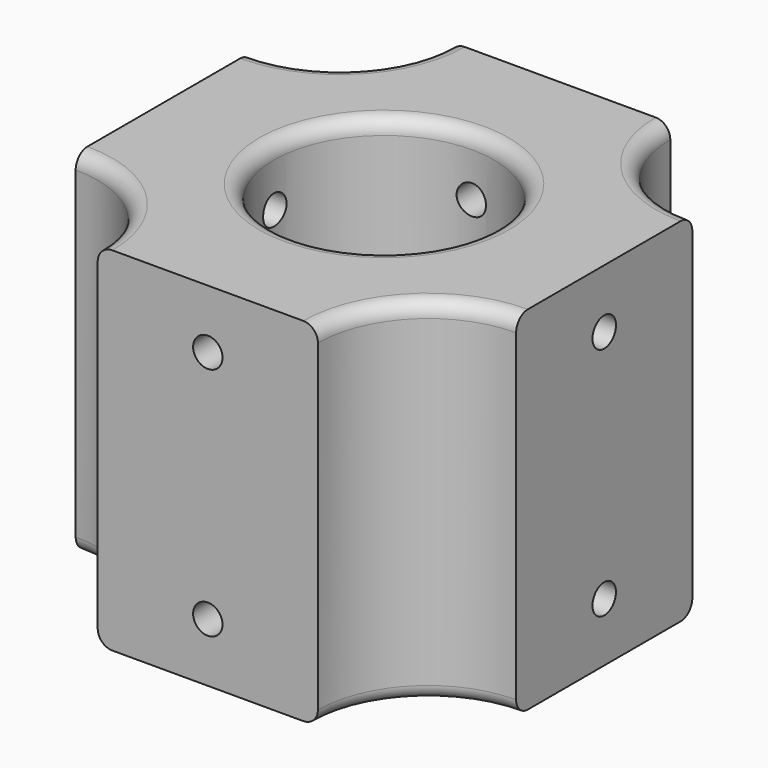
from build123d import *

# Parameters (mm, degrees)
F0_W     = 15
F0_H     = 7.5
F0_W_2   = 7.5
F0_H_2   = 15
F1_DEPTH = 12
F3_D     = 2
F5_D     = 15
F7_D     = 2
F8_R     = 1


with BuildPart() as f1:
    # F0 (on Top) → F1 (new body, symmetric)
    with BuildSketch(Plane.XY):
        with BuildLine():
            Line((-15, 7.5), (-7.5, 7.5))
            Line((-7.5, 7.5), (-7.5, 15))
            ThreePointArc((-7.5, 15), (-9.6966991411, 9.6966991411), (-15, 7.5))
        make_face()
        with Locations((0, 11.25)):
            Rectangle(F0_W, F0_H)
        with BuildLine():
            Line((7.5, 7.5), (15, 7.5))
            ThreePointArc((15, 7.5), (9.6966991411, 9.6966991411), (7.5, 15))
            Line((7.5, 15), (7.5, 7.5))
        make_face()
        with Locations((11.25, 0)):
            Rectangle(F0_W_2, F0_H_2)
        with Locations((0, -11.25)):
            Rectangle(F0_W, F0_H)
        with BuildLine():
            ThreePointArc((7.5, -15), (9.6966991411, -9.6966991411), (15, -7.5))
            Line((15, -7.5), (7.5, -7.5))
            Line((7.5, -7.5), (7.5, -15))
        make_face()
        with BuildLine():
            Line((-7.5, -15), (-7.5, -7.5))
            Line((-7.5, -7.5), (-15, -7.5))
            ThreePointArc((-15, -7.5), (-9.6966991411, -9.6966991411), (-7.5, -15))
        make_face()
        with Locations((-11.25, 0)):
            Rectangle(F0_W_2, F0_H_2)
        Rectangle(F0_W, F0_H_2)
    extrude(amount=F1_DEPTH, both=True)

    # F3 (through all)
    with Locations(Plane.XZ.offset(15)):
        with Locations((0, 8), (0, -8)):
            Hole(F3_D / 2)

    # F5 (through all)
    with Locations(Plane.XY.offset(12)):
        with Locations((0, 0)):
            Hole(F5_D / 2)

    # F7 (through all)
    with Locations(Plane(origin=(-15, 0, 0), x_dir=(0, -1, 0), z_dir=(-1, 0, 0))):
        with Locations((0, -8), (0, 8)):
            Hole(F7_D / 2)

    # F8
    f8_edges = [f1.edges().sort_by_distance(p)[0] for p in [
        (-9.696699, 9.696699, 12),
        (-9.696699, -9.696699, 12),
        (9.696699, -9.696699, 12),
        (9.696699, 9.696699, 12),
        (-9.696699, -9.696699, -12),
        (9.696699, -9.696699, -12),
        (9.696699, 9.696699, -12),
        (-9.696699, 9.696699, -12),
        (-7.5, 0, -12),
        (-7.5, 0, 12),
    ]]
    fillet(f8_edges, radius=F8_R)


solid = f1.part
